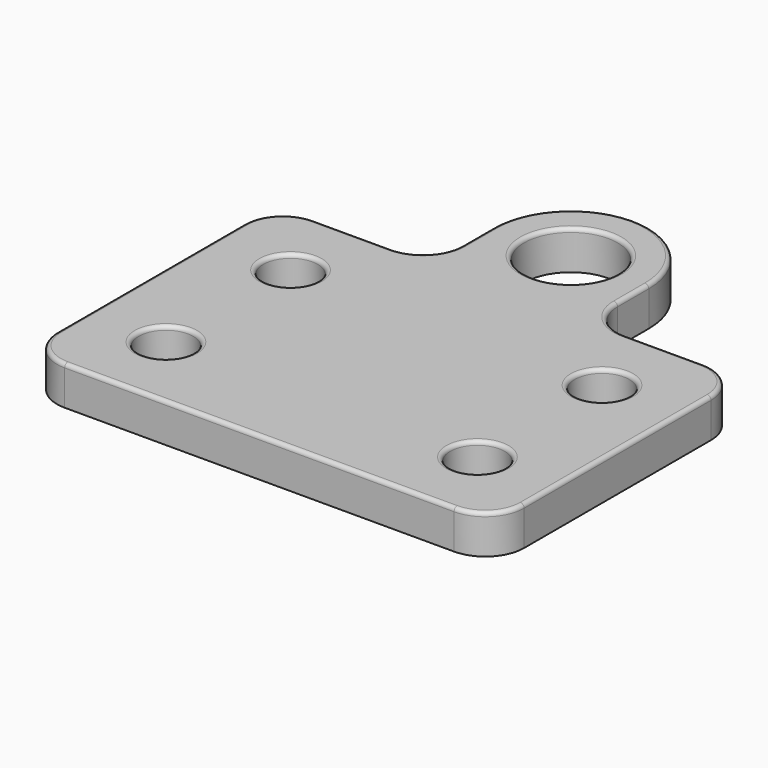
from build123d import *

# Parameters (mm, degrees)
F1_DEPTH = 5
F2_R     = 5
F4_D     = 7
F6_D     = 12
F7_R     = 0.5
F8_T     = -1
F9_R     = 0.5


with BuildPart() as f1:
    # F0 (on Top) → F1 (new body)
    with BuildSketch(Plane.XY):
        with BuildLine():
            Line((30, -20), (30, 20))
            Line((30, 20), (10, 20))
            Line((10, 20), (10, 30))
            ThreePointArc((10, 30), (0, 40), (-10, 30))
            Line((-10, 30), (-10, 20))
            Line((-10, 20), (-30, 20))
            Line((-30, 20), (-30, -20))
            Line((-30, -20), (30, -20))
        make_face()
    extrude(amount=F1_DEPTH)

    # F2
    f2_edges = [f1.edges().sort_by_distance(p)[0] for p in [
        (30, 20, 2.5),
        (30, -20, 2.5),
        (10, 20, 2.5),
        (-30, -20, 2.5),
        (-30, 20, 2.5),
        (-10, 20, 2.5),
    ]]
    fillet(f2_edges, radius=F2_R)

    # F4 (through all)
    with Locations(Plane.XY.offset(5)):
        with Locations((20, 10), (20, -10), (-20, 10), (-20, -10)):
            Hole(F4_D / 2)

    # F6 (through all)
    with Locations(Plane.XY.offset(5)):
        with Locations((0, 30)):
            Hole(F6_D / 2)

    # F7
    f7_edges = [f1.edges().sort_by_distance(p)[0] for p in [
        (30, 0, 5),
        (28.535534, -18.535534, 5),
        (28.535534, 18.535534, 5),
        (0, -20, 5),
        (20, 20, 5),
        (-28.535534, -18.535534, 5),
        (11.464466, 21.464466, 5),
        (-30, 0, 5),
        (10, 27.5, 5),
        (-28.535534, 18.535534, 5),
        (0, 40, 5),
        (-20, 20, 5),
        (-10, 27.5, 5),
        (-11.464466, 21.464466, 5),
        (-23.5, -10, 5),
        (-23.5, 10, 5),
        (16.5, -10, 5),
        (16.5, 10, 5),
        (-6, 30, 5),
    ]]
    fillet(f7_edges, radius=F7_R)

    # F8
    f8_openings = [f1.faces().sort_by_distance(p)[0] for p in [
        (0, 2.90916, 0),
    ]]
    offset(amount=F8_T, openings=f8_openings)

    # F9
    f9_edges = [f1.edges().sort_by_distance(p)[0] for p in [
        (9, 30, 2),
        (-9, 30, 2),
        (29, 0, 4),
        (27.828427, -17.828427, 4),
        (27.828427, 17.828427, 4),
        (0, -19, 4),
        (20, 19, 4),
        (-27.828427, -17.828427, 4),
        (10.757359, 20.757359, 4),
        (-29, 0, 4),
        (9, 27.5, 4),
        (-27.828427, 17.828427, 4),
        (0, 39, 4),
        (-20, 19, 4),
        (-9, 27.5, 4),
        (-10.757359, 20.757359, 4),
        (-24.5, -10, 4),
        (-24.5, 10, 4),
        (15.5, -10, 4),
        (15.5, 10, 4),
        (-7, 30, 4),
    ]]
    fillet(f9_edges, radius=F9_R)


solid = f1.part
